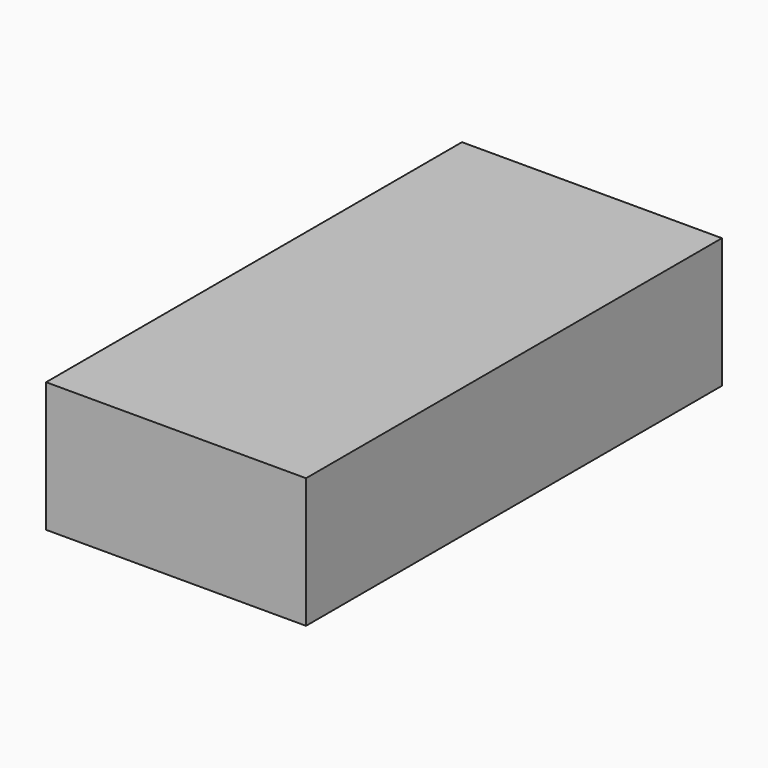
from build123d import *

# Parameters (mm, degrees)
F0_W     = 50.8
F0_H     = 25.4
F1_DEPTH = 101.6
F2_DEPTH = 130


# Not quite as in the source:
# - an extrude ends at something that could not be found from the text; its depth is read off the source's solid


with BuildPart() as f1:
    # F0 (on Front) → F1 (new body)
    with BuildSketch(Plane.XZ):
        with Locations((25.4, -12.7)):
            Rectangle(F0_W, F0_H)
    extrude(amount=F1_DEPTH)

    # F2 (cut, through all): a face of the model
    f2_faces = [f1.faces().sort_by_distance(p)[0] for p in [
        (25.4, -50.8, -25.4),
    ]]
    extrude(f2_faces, amount=F2_DEPTH, mode=Mode.SUBTRACT)


solid = f1.part
